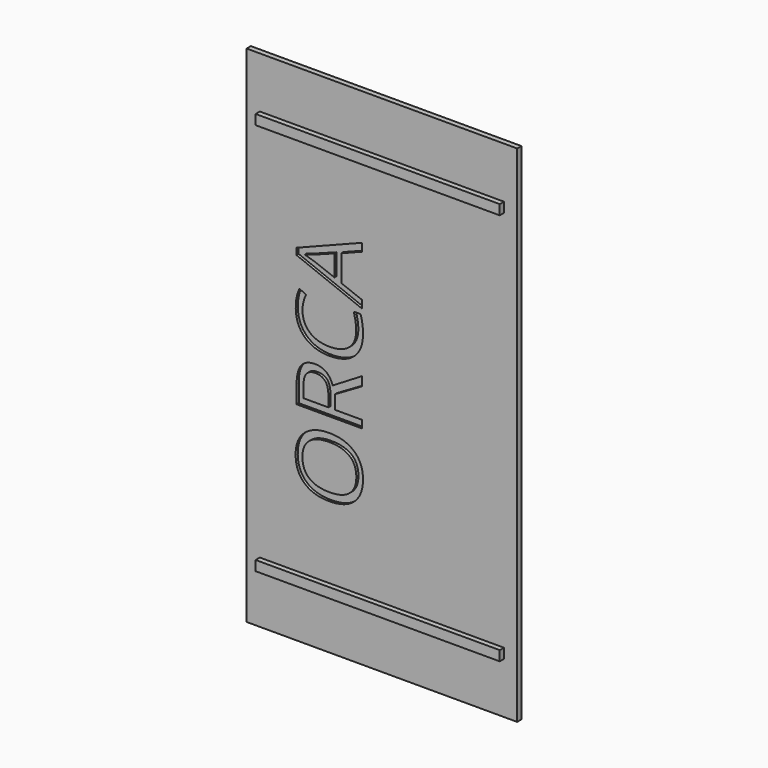
from build123d import *

# Parameters (mm, degrees)
F0_W         = 82
F0_H         = 153
F1_DEPTH     = 1.6
F3_W         = 74
F3_H         = 3
F4_DEPTH     = 1.6
F5_TEXT_SIZE = 27.7777777778
F6_DEPTH     = 0.8


# Not quite as in the source:
# - Text() gives the source's letters only with a copy of the font that has no kerning and outlines rounded to 1/6400 em; it was checked with that copy


with BuildPart() as f1:
    # F0 (on Front) → F1 (new body)
    with BuildSketch(Plane.XZ):
        with Locations((-41, 0)):
            Rectangle(F0_W, F0_H)
    extrude(amount=F1_DEPTH)

    # F3 (on offset) → F4 (join)
    with BuildSketch(Plane.XZ.offset(1.6)):
        with Locations((-41, 59.5)):
            Rectangle(F3_W, F3_H)
        with Locations((-41, -59.5)):
            Rectangle(F3_W, F3_H)
    extrude(amount=F4_DEPTH)

    # F5 (on face) → F6 (cut)
    with BuildSketch(Plane.XZ.offset(1.6)):
        with Locations(Location((-47, -37.8537326389), (0, 0, 90))):
            Text('ORCA', F5_TEXT_SIZE, font='Open Sans', text_align=(TextAlign.LEFT, TextAlign.BOTTOM))
    extrude(amount=-F6_DEPTH, mode=Mode.SUBTRACT)


solid = f1.part
